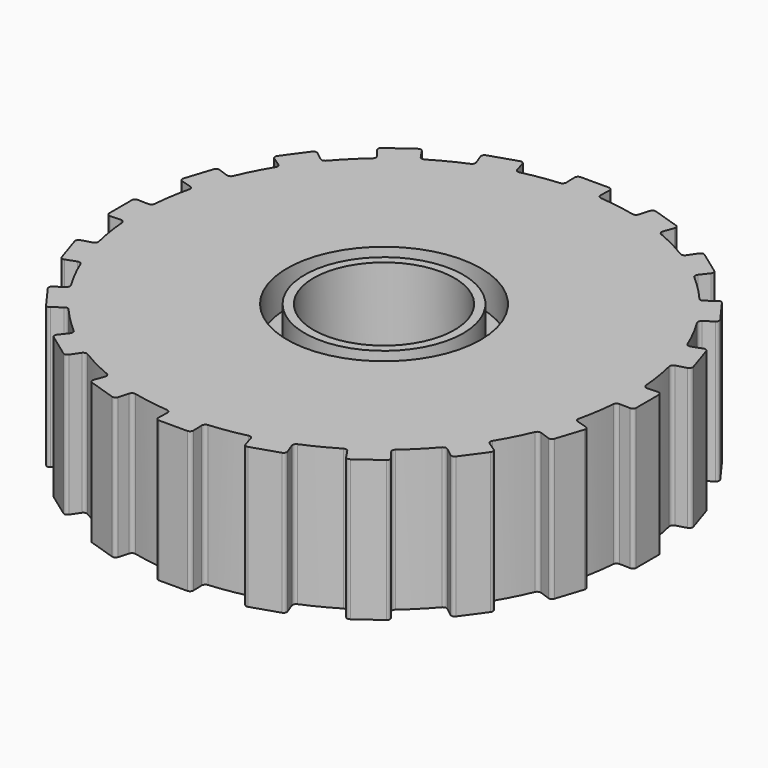
from build123d import *

# Parameters (mm, degrees)
F0_W     = 2.75
F0_H     = 2
F3_DEPTH = 25
F5_R     = 1.375
F5_R_2   = 1.125
F6_DEPTH = 0.5
F4_R     = 1.375
F4_R_2   = 1.125
F7_DEPTH = 0.5


with BuildPart() as f1:
    # F0 (on Front) → F1 (revolve)
    with BuildSketch(Plane.XZ):
        with Locations((-2.375, 1)):
            Rectangle(F0_W, F0_H)
    revolve(axis=Axis((0, 0, 1), (0, 0, 1)))

    # F2 (on face) → F3 (cut)
    with BuildSketch(Plane.XY.offset(2)):
        with BuildLine():
            ThreePointArc((-0.8032347269, 3.4065839155), (-0.5475206276, 3.4569091921), (-0.2887707016, 3.4880670122))
            Line((-0.2887707016, 3.4880670122), (-0.2983296172, 3.6916573868))
            Line((-0.2983296172, 3.6916573868), (-0.2483296172, 3.6916573868))
            Line((-0.2483296172, 3.6916573868), (-0.25, 3.7416573868))
            ThreePointArc((-0.25, 3.7416573868), (-0.5866292439, 3.7038312772), (-0.9184715906, 3.635781888))
            Line((-0.9184715906, 3.635781888), (-0.9046093693, 3.5877128856))
            Line((-0.9046093693, 3.5877128856), (-0.8630211073, 3.4435003366))
            ThreePointArc((-0.8630211073, 3.4435003366), (-0.8402539074, 3.4135015391), (-0.8032347269, 3.4065839155))
        make_face()
        with BuildLine():
            ThreePointArc((-0.2887707016, 3.4880670122), (-0.2557010319, 3.5060856191), (-0.2433182764, 3.5416516227))
            Line((-0.2433182764, 3.5416516227), (-0.2483296172, 3.6916573868))
            Line((-0.2483296172, 3.6916573868), (-0.2983296172, 3.6916573868))
            Line((-0.2983296172, 3.6916573868), (-0.2887707016, 3.4880670122))
        make_face()
        with BuildLine():
            ThreePointArc((-0.2483296172, 3.6916573868), (-0.2347697854, 3.7269080761), (-0.2, 3.7416573868))
            Line((-0.2, 3.7416573868), (-0.25, 3.7416573868))
            Line((-0.25, 3.7416573868), (-0.2483296172, 3.6916573868))
        make_face()
        with BuildLine():
            Line((-0.2, 3.7416573868), (0, 3.7416573868))
            Line((0, 3.7416573868), (0, 3.75))
            ThreePointArc((0, 3.75), (-0.1250695798, 3.7479137664), (-0.25, 3.7416573868))
            Line((-0.25, 3.7416573868), (-0.2, 3.7416573868))
        make_face()
        with BuildLine():
            Line((0, 3.75), (0, 3.7416573868))
            Line((0, 3.7416573868), (0.2, 3.7416573868))
            Line((0.2, 3.7416573868), (0.25, 3.7416573868))
            ThreePointArc((0.25, 3.7416573868), (0.1250695798, 3.7479137664), (0, 3.75))
        make_face()
        with BuildLine():
            Line((0.25, 3.7416573868), (0.2, 3.7416573868))
            ThreePointArc((0.2, 3.7416573868), (0.2347697854, 3.7269080761), (0.2483296172, 3.6916573868))
            Line((0.2483296172, 3.6916573868), (0.25, 3.7416573868))
        make_face()
        with BuildLine():
            Line((0.2983296172, 3.6916573868), (0.2887707016, 3.4880670122))
            ThreePointArc((0.2887707016, 3.4880670122), (0.5475206276, 3.4569091921), (0.8032347269, 3.4065839155))
            ThreePointArc((0.8032347269, 3.4065839155), (0.8402539074, 3.4135015391), (0.8630211073, 3.4435003366))
            Line((0.8630211073, 3.4435003366), (0.9046093693, 3.5877128856))
            Line((0.9046093693, 3.5877128856), (0.9184715906, 3.635781888))
            ThreePointArc((0.9184715906, 3.635781888), (0.5866292439, 3.7038312772), (0.25, 3.7416573868))
            Line((0.25, 3.7416573868), (0.2483296172, 3.6916573868))
            Line((0.2483296172, 3.6916573868), (0.2983296172, 3.6916573868))
        make_face()
        with BuildLine():
            Line((0.2483296172, 3.6916573868), (0.2433182764, 3.5416516227))
            ThreePointArc((0.2433182764, 3.5416516227), (0.2557010319, 3.5060856191), (0.2887707016, 3.4880670122))
            Line((0.2887707016, 3.4880670122), (0.2983296172, 3.6916573868))
            Line((0.2983296172, 3.6916573868), (0.2483296172, 3.6916573868))
        make_face()
        with BuildLine():
            Line((-2.8801181, -2.4015452797), (-2.8406490766, -2.370804649))
            ThreePointArc((-2.8406490766, -2.370804649), (-2.8771377525, -2.3805543499), (-2.9095073626, -2.36109443))
            Line((-2.9095073626, -2.36109443), (-2.8801181, -2.4015452797))
        make_face()
        with BuildLine():
            Line((-2.9095073626, -2.36109443), (-3.1446214635, -2.0374876322))
            Line((-3.1446214635, -2.0374876322), (-3.1740107261, -1.9970367825))
            ThreePointArc((-3.1740107261, -1.9970367825), (-3.0338137289, -2.2041946961), (-2.8801181, -2.4015452797))
            Line((-2.8801181, -2.4015452797), (-2.9095073626, -2.36109443))
        make_face()
        with BuildLine():
            ThreePointArc((-3.1446214635, -2.0374876322), (-3.1531261876, -2.0006888577), (-3.13257805, -1.9689988879))
            Line((-3.13257805, -1.9689988879), (-3.1740107261, -1.9970367825))
            Line((-3.1740107261, -1.9970367825), (-3.1446214635, -2.0374876322))
        make_face()
        with BuildLine():
            ThreePointArc((-2.9916406501, -1.8166139438), (-3.1185228347, -1.5889667491), (-3.228113807, -1.3525092417))
            ThreePointArc((-3.228113807, -1.3525092417), (-3.2554696104, -1.3266261727), (-3.2931213717, -1.3258399719))
            Line((-3.2931213717, -1.3258399719), (-3.4342367417, -1.3769603706))
            Line((-3.4342367417, -1.3769603706), (-3.4812733908, -1.3939998487))
            ThreePointArc((-3.4812733908, -1.3939998487), (-3.3412744657, -1.702464374), (-3.1740107261, -1.9970367825))
            Line((-3.1740107261, -1.9970367825), (-3.13257805, -1.9689988879))
            Line((-3.13257805, -1.9689988879), (-3.0082752454, -1.8848819719))
            ThreePointArc((-3.0082752454, -1.8848819719), (-2.9867801452, -1.8539589399), (-2.9916406501, -1.8166139438))
        make_face()
        with BuildLine():
            Line((-3.4812733908, -1.3939998487), (-3.4342367417, -1.3769603706))
            ThreePointArc((-3.4342367417, -1.3769603706), (-3.471952358, -1.3749572662), (-3.4967242406, -1.3464470229))
            Line((-3.4967242406, -1.3464470229), (-3.4812733908, -1.3939998487))
        make_face()
        with BuildLine():
            Line((-3.4967242406, -1.3464470229), (-3.6203310383, -0.9660244164))
            Line((-3.6203310383, -0.9660244164), (-3.635781888, -0.9184715906))
            ThreePointArc((-3.635781888, -0.9184715906), (-3.5664619361, -1.1588137289), (-3.4812733908, -1.3939998487))
            Line((-3.4812733908, -1.3939998487), (-3.4967242406, -1.3464470229))
        make_face()
        with BuildLine():
            ThreePointArc((-3.4065839155, -0.8032347269), (-3.4569091921, -0.5475206276), (-3.4880670122, -0.2887707016))
            ThreePointArc((-3.4880670122, -0.2887707016), (-3.5060856191, -0.2557010319), (-3.5416516227, -0.2433182764))
            Line((-3.5416516227, -0.2433182764), (-3.6916573868, -0.2483296172))
            Line((-3.6916573868, -0.2483296172), (-3.7416573868, -0.25))
            ThreePointArc((-3.7416573868, -0.25), (-3.7038312772, -0.5866292439), (-3.635781888, -0.9184715906))
            Line((-3.635781888, -0.9184715906), (-3.5877128856, -0.9046093693))
            Line((-3.5877128856, -0.9046093693), (-3.4435003366, -0.8630211073))
            ThreePointArc((-3.4435003366, -0.8630211073), (-3.4135015391, -0.8402539074), (-3.4065839155, -0.8032347269))
        make_face()
        with BuildLine():
            ThreePointArc((-3.6203310383, -0.9660244164), (-3.6170480649, -0.9283985978), (-3.5877128856, -0.9046093693))
            Line((-3.5877128856, -0.9046093693), (-3.635781888, -0.9184715906))
            Line((-3.635781888, -0.9184715906), (-3.6203310383, -0.9660244164))
        make_face()
        with BuildLine():
            Line((-3.7416573868, -0.2), (-3.7416573868, 0.2))
            Line((-3.7416573868, 0.2), (-3.7416573868, 0.25))
            ThreePointArc((-3.7416573868, 0.25), (-3.75, 0), (-3.7416573868, -0.25))
            Line((-3.7416573868, -0.25), (-3.7416573868, -0.2))
        make_face()
        with BuildLine():
            Line((-3.7416573868, -0.25), (-3.6916573868, -0.2483296172))
            ThreePointArc((-3.6916573868, -0.2483296172), (-3.7269080761, -0.2347697854), (-3.7416573868, -0.2))
            Line((-3.7416573868, -0.2), (-3.7416573868, -0.25))
        make_face()
        with BuildLine():
            ThreePointArc((-3.7416573868, 0.2), (-3.7269080761, 0.2347697854), (-3.6916573868, 0.2483296172))
            Line((-3.6916573868, 0.2483296172), (-3.7416573868, 0.25))
            Line((-3.7416573868, 0.25), (-3.7416573868, 0.2))
        make_face()
        with BuildLine():
            ThreePointArc((-3.4880670122, 0.2887707016), (-3.4569091921, 0.5475206276), (-3.4065839155, 0.8032347269))
            ThreePointArc((-3.4065839155, 0.8032347269), (-3.4135015391, 0.8402539074), (-3.4435003366, 0.8630211073))
            Line((-3.4435003366, 0.8630211073), (-3.5877128856, 0.9046093693))
            Line((-3.5877128856, 0.9046093693), (-3.635781888, 0.9184715906))
            ThreePointArc((-3.635781888, 0.9184715906), (-3.7038312772, 0.5866292439), (-3.7416573868, 0.25))
            Line((-3.7416573868, 0.25), (-3.6916573868, 0.2483296172))
            Line((-3.6916573868, 0.2483296172), (-3.5416516227, 0.2433182764))
            ThreePointArc((-3.5416516227, 0.2433182764), (-3.5060856191, 0.2557010319), (-3.4880670122, 0.2887707016))
        make_face()
        with BuildLine():
            Line((-3.635781888, 0.9184715906), (-3.5877128856, 0.9046093693))
            ThreePointArc((-3.5877128856, 0.9046093693), (-3.6170480649, 0.9283985978), (-3.6203310383, 0.9660244164))
            Line((-3.6203310383, 0.9660244164), (-3.635781888, 0.9184715906))
        make_face()
        with BuildLine():
            Line((-3.6203310383, 0.9660244164), (-3.4967242406, 1.3464470229))
            Line((-3.4967242406, 1.3464470229), (-3.4812733908, 1.3939998487))
            ThreePointArc((-3.4812733908, 1.3939998487), (-3.5664619361, 1.1588137289), (-3.635781888, 0.9184715906))
            Line((-3.635781888, 0.9184715906), (-3.6203310383, 0.9660244164))
        make_face()
        with BuildLine():
            ThreePointArc((-3.4967242406, 1.3464470229), (-3.471952358, 1.3749572662), (-3.4342367417, 1.3769603706))
            Line((-3.4342367417, 1.3769603706), (-3.4812733908, 1.3939998487))
            Line((-3.4812733908, 1.3939998487), (-3.4967242406, 1.3464470229))
        make_face()
        with BuildLine():
            ThreePointArc((-3.228113807, 1.3525092417), (-3.1185228347, 1.5889667491), (-2.9916406501, 1.8166139438))
            ThreePointArc((-2.9916406501, 1.8166139438), (-2.9867801452, 1.8539589399), (-3.0082752454, 1.8848819719))
            Line((-3.0082752454, 1.8848819719), (-3.13257805, 1.9689988879))
            Line((-3.13257805, 1.9689988879), (-3.1740107261, 1.9970367825))
            ThreePointArc((-3.1740107261, 1.9970367825), (-3.3412744657, 1.702464374), (-3.4812733908, 1.3939998487))
            Line((-3.4812733908, 1.3939998487), (-3.4342367417, 1.3769603706))
            Line((-3.4342367417, 1.3769603706), (-3.2931213717, 1.3258399719))
            ThreePointArc((-3.2931213717, 1.3258399719), (-3.2554696104, 1.3266261727), (-3.228113807, 1.3525092417))
        make_face()
        with BuildLine():
            Line((-3.1740107261, 1.9970367825), (-3.13257805, 1.9689988879))
            ThreePointArc((-3.13257805, 1.9689988879), (-3.1531261876, 2.0006888577), (-3.1446214635, 2.0374876322))
            Line((-3.1446214635, 2.0374876322), (-3.1740107261, 1.9970367825))
        make_face()
        with BuildLine():
            Line((-3.1446214635, 2.0374876322), (-2.9095073626, 2.36109443))
            Line((-2.9095073626, 2.36109443), (-2.8801181, 2.4015452797))
            ThreePointArc((-2.8801181, 2.4015452797), (-3.0338137289, 2.2041946961), (-3.1740107261, 1.9970367825))
            Line((-3.1740107261, 1.9970367825), (-3.1446214635, 2.0374876322))
        make_face()
        with BuildLine():
            ThreePointArc((-2.9095073626, 2.36109443), (-2.8771377525, 2.3805543499), (-2.8406490766, 2.370804649))
            Line((-2.8406490766, 2.370804649), (-2.8801181, 2.4015452797))
            Line((-2.8801181, 2.4015452797), (-2.9095073626, 2.36109443))
        make_face()
        with BuildLine():
            Line((-2.36109443, 2.9095073626), (-2.0374876322, 3.1446214635))
            Line((-2.0374876322, 3.1446214635), (-1.9970367825, 3.1740107261))
            ThreePointArc((-1.9970367825, 3.1740107261), (-2.2041946961, 3.0338137289), (-2.4015452797, 2.8801181))
            Line((-2.4015452797, 2.8801181), (-2.36109443, 2.9095073626))
        make_face()
        with BuildLine():
            Line((-2.4015452797, 2.8801181), (-2.370804649, 2.8406490766))
            ThreePointArc((-2.370804649, 2.8406490766), (-2.3805543499, 2.8771377525), (-2.36109443, 2.9095073626))
            Line((-2.36109443, 2.9095073626), (-2.4015452797, 2.8801181))
        make_face()
        with BuildLine():
            ThreePointArc((-2.6521703308, 2.2838547538), (-2.4748737342, 2.4748737342), (-2.2838547538, 2.6521703308))
            ThreePointArc((-2.2838547538, 2.6521703308), (-2.2676919005, 2.686185554), (-2.2785792132, 2.7222374564))
            Line((-2.2785792132, 2.7222374564), (-2.370804649, 2.8406490766))
            Line((-2.370804649, 2.8406490766), (-2.4015452797, 2.8801181))
            ThreePointArc((-2.4015452797, 2.8801181), (-2.6516504294, 2.6516504294), (-2.8801181, 2.4015452797))
            Line((-2.8801181, 2.4015452797), (-2.8406490766, 2.370804649))
            Line((-2.8406490766, 2.370804649), (-2.7222374564, 2.2785792132))
            ThreePointArc((-2.7222374564, 2.2785792132), (-2.686185554, 2.2676919005), (-2.6521703308, 2.2838547538))
        make_face()
        with BuildLine():
            ThreePointArc((-2.0374876322, 3.1446214635), (-2.0006888577, 3.1531261876), (-1.9689988879, 3.13257805))
            Line((-1.9689988879, 3.13257805), (-1.9970367825, 3.1740107261))
            Line((-1.9970367825, 3.1740107261), (-2.0374876322, 3.1446214635))
        make_face()
        with BuildLine():
            ThreePointArc((-1.8166139438, 2.9916406501), (-1.5889667491, 3.1185228347), (-1.3525092417, 3.228113807))
            ThreePointArc((-1.3525092417, 3.228113807), (-1.3266261727, 3.2554696104), (-1.3258399719, 3.2931213717))
            Line((-1.3258399719, 3.2931213717), (-1.3769603706, 3.4342367417))
            Line((-1.3769603706, 3.4342367417), (-1.3939998487, 3.4812733908))
            ThreePointArc((-1.3939998487, 3.4812733908), (-1.702464374, 3.3412744657), (-1.9970367825, 3.1740107261))
            Line((-1.9970367825, 3.1740107261), (-1.9689988879, 3.13257805))
            Line((-1.9689988879, 3.13257805), (-1.8848819719, 3.0082752454))
            ThreePointArc((-1.8848819719, 3.0082752454), (-1.8539589399, 2.9867801452), (-1.8166139438, 2.9916406501))
        make_face()
        with BuildLine():
            Line((-1.3939998487, 3.4812733908), (-1.3769603706, 3.4342367417))
            ThreePointArc((-1.3769603706, 3.4342367417), (-1.3749572662, 3.471952358), (-1.3464470229, 3.4967242406))
            Line((-1.3464470229, 3.4967242406), (-1.3939998487, 3.4812733908))
        make_face()
        with BuildLine():
            ThreePointArc((-0.9660244164, 3.6203310383), (-0.9283985978, 3.6170480649), (-0.9046093693, 3.5877128856))
            Line((-0.9046093693, 3.5877128856), (-0.9184715906, 3.635781888))
            Line((-0.9184715906, 3.635781888), (-0.9660244164, 3.6203310383))
        make_face()
        with BuildLine():
            Line((-0.9660244164, 3.6203310383), (-0.9184715906, 3.635781888))
            ThreePointArc((-0.9184715906, 3.635781888), (-1.1588137289, 3.5664619361), (-1.3939998487, 3.4812733908))
            Line((-1.3939998487, 3.4812733908), (-1.3464470229, 3.4967242406))
            Line((-1.3464470229, 3.4967242406), (-0.9660244164, 3.6203310383))
        make_face()
        with BuildLine():
            Line((3.1740107261, -1.9970367825), (3.13257805, -1.9689988879))
            ThreePointArc((3.13257805, -1.9689988879), (3.1531261876, -2.0006888577), (3.1446214635, -2.0374876322))
            Line((3.1446214635, -2.0374876322), (3.1740107261, -1.9970367825))
        make_face()
        with BuildLine():
            ThreePointArc((2.8801181, -2.4015452797), (3.0338137289, -2.2041946961), (3.1740107261, -1.9970367825))
            Line((3.1740107261, -1.9970367825), (3.1446214635, -2.0374876322))
            Line((3.1446214635, -2.0374876322), (2.9095073626, -2.36109443))
            Line((2.9095073626, -2.36109443), (2.8801181, -2.4015452797))
        make_face()
        with BuildLine():
            ThreePointArc((2.9095073626, -2.36109443), (2.8771377525, -2.3805543499), (2.8406490766, -2.370804649))
            Line((2.8406490766, -2.370804649), (2.8801181, -2.4015452797))
            Line((2.8801181, -2.4015452797), (2.9095073626, -2.36109443))
        make_face()
        with BuildLine():
            ThreePointArc((2.6521703308, -2.2838547538), (2.4748737342, -2.4748737342), (2.2838547538, -2.6521703308))
            ThreePointArc((2.2838547538, -2.6521703308), (2.2676919005, -2.686185554), (2.2785792132, -2.7222374564))
            Line((2.2785792132, -2.7222374564), (2.370804649, -2.8406490766))
            Line((2.370804649, -2.8406490766), (2.4015452797, -2.8801181))
            ThreePointArc((2.4015452797, -2.8801181), (2.6516504294, -2.6516504294), (2.8801181, -2.4015452797))
            Line((2.8801181, -2.4015452797), (2.8406490766, -2.370804649))
            Line((2.8406490766, -2.370804649), (2.7222374564, -2.2785792132))
            ThreePointArc((2.7222374564, -2.2785792132), (2.686185554, -2.2676919005), (2.6521703308, -2.2838547538))
        make_face()
        with BuildLine():
            Line((2.4015452797, -2.8801181), (2.370804649, -2.8406490766))
            ThreePointArc((2.370804649, -2.8406490766), (2.3805543499, -2.8771377525), (2.36109443, -2.9095073626))
            Line((2.36109443, -2.9095073626), (2.4015452797, -2.8801181))
        make_face()
        with BuildLine():
            ThreePointArc((1.9970367825, -3.1740107261), (2.2041946961, -3.0338137289), (2.4015452797, -2.8801181))
            Line((2.4015452797, -2.8801181), (2.36109443, -2.9095073626))
            Line((2.36109443, -2.9095073626), (2.0374876322, -3.1446214635))
            Line((2.0374876322, -3.1446214635), (1.9970367825, -3.1740107261))
        make_face()
        with BuildLine():
            ThreePointArc((2.0374876322, -3.1446214635), (2.0006888577, -3.1531261876), (1.9689988879, -3.13257805))
            Line((1.9689988879, -3.13257805), (1.9970367825, -3.1740107261))
            Line((1.9970367825, -3.1740107261), (2.0374876322, -3.1446214635))
        make_face()
        with BuildLine():
            ThreePointArc((1.8166139438, -2.9916406501), (1.5889667491, -3.1185228347), (1.3525092417, -3.228113807))
            ThreePointArc((1.3525092417, -3.228113807), (1.3266261727, -3.2554696104), (1.3258399719, -3.2931213717))
            Line((1.3258399719, -3.2931213717), (1.3769603706, -3.4342367417))
            Line((1.3769603706, -3.4342367417), (1.3939998487, -3.4812733908))
            ThreePointArc((1.3939998487, -3.4812733908), (1.702464374, -3.3412744657), (1.9970367825, -3.1740107261))
            Line((1.9970367825, -3.1740107261), (1.9689988879, -3.13257805))
            Line((1.9689988879, -3.13257805), (1.8848819719, -3.0082752454))
            ThreePointArc((1.8848819719, -3.0082752454), (1.8539589399, -2.9867801452), (1.8166139438, -2.9916406501))
        make_face()
        with BuildLine():
            Line((1.3939998487, -3.4812733908), (1.3769603706, -3.4342367417))
            ThreePointArc((1.3769603706, -3.4342367417), (1.3749572662, -3.471952358), (1.3464470229, -3.4967242406))
            Line((1.3464470229, -3.4967242406), (1.3939998487, -3.4812733908))
        make_face()
        with BuildLine():
            ThreePointArc((0.9184715906, -3.635781888), (1.1588137289, -3.5664619361), (1.3939998487, -3.4812733908))
            Line((1.3939998487, -3.4812733908), (1.3464470229, -3.4967242406))
            Line((1.3464470229, -3.4967242406), (0.9660244164, -3.6203310383))
            Line((0.9660244164, -3.6203310383), (0.9184715906, -3.635781888))
        make_face()
        with BuildLine():
            Line((0.25, -3.7416573868), (0.2483296172, -3.6916573868))
            ThreePointArc((0.2483296172, -3.6916573868), (0.2347697854, -3.7269080761), (0.2, -3.7416573868))
            Line((0.2, -3.7416573868), (0.25, -3.7416573868))
        make_face()
        with BuildLine():
            ThreePointArc((-0.25, -3.7416573868), (0, -3.75), (0.25, -3.7416573868))
            Line((0.25, -3.7416573868), (0.2, -3.7416573868))
            Line((0.2, -3.7416573868), (-0.2, -3.7416573868))
            Line((-0.2, -3.7416573868), (-0.25, -3.7416573868))
        make_face()
        with BuildLine():
            Line((-0.9184715906, -3.635781888), (-0.9046093693, -3.5877128856))
            ThreePointArc((-0.9046093693, -3.5877128856), (-0.9283985978, -3.6170480649), (-0.9660244164, -3.6203310383))
            Line((-0.9660244164, -3.6203310383), (-0.9184715906, -3.635781888))
        make_face()
        with BuildLine():
            Line((-0.9660244164, -3.6203310383), (-1.3464470229, -3.4967242406))
            Line((-1.3464470229, -3.4967242406), (-1.3939998487, -3.4812733908))
            ThreePointArc((-1.3939998487, -3.4812733908), (-1.1588137289, -3.5664619361), (-0.9184715906, -3.635781888))
            Line((-0.9184715906, -3.635781888), (-0.9660244164, -3.6203310383))
        make_face()
        with BuildLine():
            ThreePointArc((-1.3464470229, -3.4967242406), (-1.3749572662, -3.471952358), (-1.3769603706, -3.4342367417))
            Line((-1.3769603706, -3.4342367417), (-1.3939998487, -3.4812733908))
            Line((-1.3939998487, -3.4812733908), (-1.3464470229, -3.4967242406))
        make_face()
        with BuildLine():
            ThreePointArc((-1.3525092417, -3.228113807), (-1.5889667491, -3.1185228347), (-1.8166139438, -2.9916406501))
            ThreePointArc((-1.8166139438, -2.9916406501), (-1.8539589399, -2.9867801452), (-1.8848819719, -3.0082752454))
            Line((-1.8848819719, -3.0082752454), (-1.9689988879, -3.13257805))
            Line((-1.9689988879, -3.13257805), (-1.9970367825, -3.1740107261))
            ThreePointArc((-1.9970367825, -3.1740107261), (-1.702464374, -3.3412744657), (-1.3939998487, -3.4812733908))
            Line((-1.3939998487, -3.4812733908), (-1.3769603706, -3.4342367417))
            Line((-1.3769603706, -3.4342367417), (-1.3258399719, -3.2931213717))
            ThreePointArc((-1.3258399719, -3.2931213717), (-1.3266261727, -3.2554696104), (-1.3525092417, -3.228113807))
        make_face()
        with BuildLine():
            ThreePointArc((-0.2887707016, -3.4880670122), (-0.5475206276, -3.4569091921), (-0.8032347269, -3.4065839155))
            ThreePointArc((-0.8032347269, -3.4065839155), (-0.8402539074, -3.4135015391), (-0.8630211073, -3.4435003366))
            Line((-0.8630211073, -3.4435003366), (-0.9046093693, -3.5877128856))
            Line((-0.9046093693, -3.5877128856), (-0.9184715906, -3.635781888))
            ThreePointArc((-0.9184715906, -3.635781888), (-0.5866292439, -3.7038312772), (-0.25, -3.7416573868))
            Line((-0.25, -3.7416573868), (-0.2483296172, -3.6916573868))
            Line((-0.2483296172, -3.6916573868), (-0.2433182764, -3.5416516227))
            ThreePointArc((-0.2433182764, -3.5416516227), (-0.2557010319, -3.5060856191), (-0.2887707016, -3.4880670122))
        make_face()
        with BuildLine():
            ThreePointArc((0.8032347269, -3.4065839155), (0.5475206276, -3.4569091921), (0.2887707016, -3.4880670122))
            ThreePointArc((0.2887707016, -3.4880670122), (0.2557010319, -3.5060856191), (0.2433182764, -3.5416516227))
            Line((0.2433182764, -3.5416516227), (0.2483296172, -3.6916573868))
            Line((0.2483296172, -3.6916573868), (0.25, -3.7416573868))
            ThreePointArc((0.25, -3.7416573868), (0.5866292439, -3.7038312772), (0.9184715906, -3.635781888))
            Line((0.9184715906, -3.635781888), (0.9046093693, -3.5877128856))
            Line((0.9046093693, -3.5877128856), (0.8630211073, -3.4435003366))
            ThreePointArc((0.8630211073, -3.4435003366), (0.8402539074, -3.4135015391), (0.8032347269, -3.4065839155))
        make_face()
        with BuildLine():
            ThreePointArc((-0.2, -3.7416573868), (-0.2347697854, -3.7269080761), (-0.2483296172, -3.6916573868))
            Line((-0.2483296172, -3.6916573868), (-0.25, -3.7416573868))
            Line((-0.25, -3.7416573868), (-0.2, -3.7416573868))
        make_face()
        with BuildLine():
            ThreePointArc((0.9660244164, -3.6203310383), (0.9283985978, -3.6170480649), (0.9046093693, -3.5877128856))
            Line((0.9046093693, -3.5877128856), (0.9184715906, -3.635781888))
            Line((0.9184715906, -3.635781888), (0.9660244164, -3.6203310383))
        make_face()
        with BuildLine():
            Line((-1.9970367825, -3.1740107261), (-1.9689988879, -3.13257805))
            ThreePointArc((-1.9689988879, -3.13257805), (-2.0006888577, -3.1531261876), (-2.0374876322, -3.1446214635))
            Line((-2.0374876322, -3.1446214635), (-1.9970367825, -3.1740107261))
        make_face()
        with BuildLine():
            Line((-2.0374876322, -3.1446214635), (-2.36109443, -2.9095073626))
            Line((-2.36109443, -2.9095073626), (-2.4015452797, -2.8801181))
            ThreePointArc((-2.4015452797, -2.8801181), (-2.2041946961, -3.0338137289), (-1.9970367825, -3.1740107261))
            Line((-1.9970367825, -3.1740107261), (-2.0374876322, -3.1446214635))
        make_face()
        with BuildLine():
            ThreePointArc((-2.36109443, -2.9095073626), (-2.3805543499, -2.8771377525), (-2.370804649, -2.8406490766))
            Line((-2.370804649, -2.8406490766), (-2.4015452797, -2.8801181))
            Line((-2.4015452797, -2.8801181), (-2.36109443, -2.9095073626))
        make_face()
        with BuildLine():
            ThreePointArc((-2.2838547538, -2.6521703308), (-2.4748737342, -2.4748737342), (-2.6521703308, -2.2838547538))
            ThreePointArc((-2.6521703308, -2.2838547538), (-2.686185554, -2.2676919005), (-2.7222374564, -2.2785792132))
            Line((-2.7222374564, -2.2785792132), (-2.8406490766, -2.370804649))
            Line((-2.8406490766, -2.370804649), (-2.8801181, -2.4015452797))
            ThreePointArc((-2.8801181, -2.4015452797), (-2.6516504294, -2.6516504294), (-2.4015452797, -2.8801181))
            Line((-2.4015452797, -2.8801181), (-2.370804649, -2.8406490766))
            Line((-2.370804649, -2.8406490766), (-2.2785792132, -2.7222374564))
            ThreePointArc((-2.2785792132, -2.7222374564), (-2.2676919005, -2.686185554), (-2.2838547538, -2.6521703308))
        make_face()
        with BuildLine():
            ThreePointArc((3.228113807, -1.3525092417), (3.1185228347, -1.5889667491), (2.9916406501, -1.8166139438))
            ThreePointArc((2.9916406501, -1.8166139438), (2.9867801452, -1.8539589399), (3.0082752454, -1.8848819719))
            Line((3.0082752454, -1.8848819719), (3.13257805, -1.9689988879))
            Line((3.13257805, -1.9689988879), (3.1740107261, -1.9970367825))
            ThreePointArc((3.1740107261, -1.9970367825), (3.3412744657, -1.702464374), (3.4812733908, -1.3939998487))
            Line((3.4812733908, -1.3939998487), (3.4342367417, -1.3769603706))
            Line((3.4342367417, -1.3769603706), (3.2931213717, -1.3258399719))
            ThreePointArc((3.2931213717, -1.3258399719), (3.2554696104, -1.3266261727), (3.228113807, -1.3525092417))
        make_face()
        with BuildLine():
            ThreePointArc((3.4967242406, -1.3464470229), (3.471952358, -1.3749572662), (3.4342367417, -1.3769603706))
            Line((3.4342367417, -1.3769603706), (3.4812733908, -1.3939998487))
            Line((3.4812733908, -1.3939998487), (3.4967242406, -1.3464470229))
        make_face()
        with BuildLine():
            ThreePointArc((3.4812733908, -1.3939998487), (3.5664619361, -1.1588137289), (3.635781888, -0.9184715906))
            Line((3.635781888, -0.9184715906), (3.6203310383, -0.9660244164))
            Line((3.6203310383, -0.9660244164), (3.4967242406, -1.3464470229))
            Line((3.4967242406, -1.3464470229), (3.4812733908, -1.3939998487))
        make_face()
        with BuildLine():
            Line((3.635781888, -0.9184715906), (3.5877128856, -0.9046093693))
            ThreePointArc((3.5877128856, -0.9046093693), (3.6170480649, -0.9283985978), (3.6203310383, -0.9660244164))
            Line((3.6203310383, -0.9660244164), (3.635781888, -0.9184715906))
        make_face()
        with BuildLine():
            ThreePointArc((3.4880670122, -0.2887707016), (3.4569091921, -0.5475206276), (3.4065839155, -0.8032347269))
            ThreePointArc((3.4065839155, -0.8032347269), (3.4135015391, -0.8402539074), (3.4435003366, -0.8630211073))
            Line((3.4435003366, -0.8630211073), (3.5877128856, -0.9046093693))
            Line((3.5877128856, -0.9046093693), (3.635781888, -0.9184715906))
            ThreePointArc((3.635781888, -0.9184715906), (3.7038312772, -0.5866292439), (3.7416573868, -0.25))
            Line((3.7416573868, -0.25), (3.6916573868, -0.2483296172))
            Line((3.6916573868, -0.2483296172), (3.5416516227, -0.2433182764))
            ThreePointArc((3.5416516227, -0.2433182764), (3.5060856191, -0.2557010319), (3.4880670122, -0.2887707016))
        make_face()
        with BuildLine():
            ThreePointArc((3.75, 0), (3.7479137664, 0.1250695798), (3.7416573868, 0.25))
            Line((3.7416573868, 0.25), (3.7416573868, 0.2))
            Line((3.7416573868, 0.2), (3.7416573868, -0.2))
            Line((3.7416573868, -0.2), (3.7416573868, -0.25))
            ThreePointArc((3.7416573868, -0.25), (3.7479137664, -0.1250695798), (3.75, 0))
        make_face()
        with BuildLine():
            Line((3.7416573868, 0.25), (3.6916573868, 0.2483296172))
            ThreePointArc((3.6916573868, 0.2483296172), (3.7269080761, 0.2347697854), (3.7416573868, 0.2))
            Line((3.7416573868, 0.2), (3.7416573868, 0.25))
        make_face()
        with BuildLine():
            ThreePointArc((3.7416573868, -0.2), (3.7269080761, -0.2347697854), (3.6916573868, -0.2483296172))
            Line((3.6916573868, -0.2483296172), (3.7416573868, -0.25))
            Line((3.7416573868, -0.25), (3.7416573868, -0.2))
        make_face()
        with BuildLine():
            ThreePointArc((3.4065839155, 0.8032347269), (3.4569091921, 0.5475206276), (3.4880670122, 0.2887707016))
            ThreePointArc((3.4880670122, 0.2887707016), (3.5060856191, 0.2557010319), (3.5416516227, 0.2433182764))
            Line((3.5416516227, 0.2433182764), (3.6916573868, 0.2483296172))
            Line((3.6916573868, 0.2483296172), (3.7416573868, 0.25))
            ThreePointArc((3.7416573868, 0.25), (3.7038312772, 0.5866292439), (3.635781888, 0.9184715906))
            Line((3.635781888, 0.9184715906), (3.5877128856, 0.9046093693))
            Line((3.5877128856, 0.9046093693), (3.4435003366, 0.8630211073))
            ThreePointArc((3.4435003366, 0.8630211073), (3.4135015391, 0.8402539074), (3.4065839155, 0.8032347269))
        make_face()
        with BuildLine():
            ThreePointArc((3.6203310383, 0.9660244164), (3.6170480649, 0.9283985978), (3.5877128856, 0.9046093693))
            Line((3.5877128856, 0.9046093693), (3.635781888, 0.9184715906))
            Line((3.635781888, 0.9184715906), (3.6203310383, 0.9660244164))
        make_face()
        with BuildLine():
            ThreePointArc((3.635781888, 0.9184715906), (3.5664619361, 1.1588137289), (3.4812733908, 1.3939998487))
            Line((3.4812733908, 1.3939998487), (3.4967242406, 1.3464470229))
            Line((3.4967242406, 1.3464470229), (3.6203310383, 0.9660244164))
            Line((3.6203310383, 0.9660244164), (3.635781888, 0.9184715906))
        make_face()
        with BuildLine():
            Line((3.4812733908, 1.3939998487), (3.4342367417, 1.3769603706))
            ThreePointArc((3.4342367417, 1.3769603706), (3.471952358, 1.3749572662), (3.4967242406, 1.3464470229))
            Line((3.4967242406, 1.3464470229), (3.4812733908, 1.3939998487))
        make_face()
        with BuildLine():
            ThreePointArc((2.9916406501, 1.8166139438), (3.1185228347, 1.5889667491), (3.228113807, 1.3525092417))
            ThreePointArc((3.228113807, 1.3525092417), (3.2554696104, 1.3266261727), (3.2931213717, 1.3258399719))
            Line((3.2931213717, 1.3258399719), (3.4342367417, 1.3769603706))
            Line((3.4342367417, 1.3769603706), (3.4812733908, 1.3939998487))
            ThreePointArc((3.4812733908, 1.3939998487), (3.3412744657, 1.702464374), (3.1740107261, 1.9970367825))
            Line((3.1740107261, 1.9970367825), (3.13257805, 1.9689988879))
            Line((3.13257805, 1.9689988879), (3.0082752454, 1.8848819719))
            ThreePointArc((3.0082752454, 1.8848819719), (2.9867801452, 1.8539589399), (2.9916406501, 1.8166139438))
        make_face()
        with BuildLine():
            ThreePointArc((3.1740107261, 1.9970367825), (3.0338137289, 2.2041946961), (2.8801181, 2.4015452797))
            Line((2.8801181, 2.4015452797), (2.9095073626, 2.36109443))
            Line((2.9095073626, 2.36109443), (3.1446214635, 2.0374876322))
            Line((3.1446214635, 2.0374876322), (3.1740107261, 1.9970367825))
        make_face()
        with BuildLine():
            ThreePointArc((3.1446214635, 2.0374876322), (3.1531261876, 2.0006888577), (3.13257805, 1.9689988879))
            Line((3.13257805, 1.9689988879), (3.1740107261, 1.9970367825))
            Line((3.1740107261, 1.9970367825), (3.1446214635, 2.0374876322))
        make_face()
        with BuildLine():
            Line((2.8801181, 2.4015452797), (2.8406490766, 2.370804649))
            ThreePointArc((2.8406490766, 2.370804649), (2.8771377525, 2.3805543499), (2.9095073626, 2.36109443))
            Line((2.9095073626, 2.36109443), (2.8801181, 2.4015452797))
        make_face()
        with BuildLine():
            ThreePointArc((2.2785792132, 2.7222374564), (2.2676919005, 2.686185554), (2.2838547538, 2.6521703308))
            ThreePointArc((2.2838547538, 2.6521703308), (2.4748737342, 2.4748737342), (2.6521703308, 2.2838547538))
            ThreePointArc((2.6521703308, 2.2838547538), (2.686185554, 2.2676919005), (2.7222374564, 2.2785792132))
            Line((2.7222374564, 2.2785792132), (2.8406490766, 2.370804649))
            Line((2.8406490766, 2.370804649), (2.8801181, 2.4015452797))
            ThreePointArc((2.8801181, 2.4015452797), (2.6516504294, 2.6516504294), (2.4015452797, 2.8801181))
            Line((2.4015452797, 2.8801181), (2.370804649, 2.8406490766))
            Line((2.370804649, 2.8406490766), (2.2785792132, 2.7222374564))
        make_face()
        with BuildLine():
            ThreePointArc((2.4015452797, 2.8801181), (2.2041946961, 3.0338137289), (1.9970367825, 3.1740107261))
            Line((1.9970367825, 3.1740107261), (2.0374876322, 3.1446214635))
            Line((2.0374876322, 3.1446214635), (2.36109443, 2.9095073626))
            Line((2.36109443, 2.9095073626), (2.4015452797, 2.8801181))
        make_face()
        with BuildLine():
            ThreePointArc((2.36109443, 2.9095073626), (2.3805543499, 2.8771377525), (2.370804649, 2.8406490766))
            Line((2.370804649, 2.8406490766), (2.4015452797, 2.8801181))
            Line((2.4015452797, 2.8801181), (2.36109443, 2.9095073626))
        make_face()
        with BuildLine():
            ThreePointArc((1.3939998487, 3.4812733908), (1.1588137289, 3.5664619361), (0.9184715906, 3.635781888))
            Line((0.9184715906, 3.635781888), (0.9660244164, 3.6203310383))
            Line((0.9660244164, 3.6203310383), (1.3464470229, 3.4967242406))
            Line((1.3464470229, 3.4967242406), (1.3939998487, 3.4812733908))
        make_face()
        with BuildLine():
            ThreePointArc((1.3464470229, 3.4967242406), (1.3749572662, 3.471952358), (1.3769603706, 3.4342367417))
            Line((1.3769603706, 3.4342367417), (1.3939998487, 3.4812733908))
            Line((1.3939998487, 3.4812733908), (1.3464470229, 3.4967242406))
        make_face()
        with BuildLine():
            Line((0.9184715906, 3.635781888), (0.9046093693, 3.5877128856))
            ThreePointArc((0.9046093693, 3.5877128856), (0.9283985978, 3.6170480649), (0.9660244164, 3.6203310383))
            Line((0.9660244164, 3.6203310383), (0.9184715906, 3.635781888))
        make_face()
        with BuildLine():
            ThreePointArc((1.3258399719, 3.2931213717), (1.3266261727, 3.2554696104), (1.3525092417, 3.228113807))
            ThreePointArc((1.3525092417, 3.228113807), (1.5889667491, 3.1185228347), (1.8166139438, 2.9916406501))
            ThreePointArc((1.8166139438, 2.9916406501), (1.8539589399, 2.9867801452), (1.8848819719, 3.0082752454))
            Line((1.8848819719, 3.0082752454), (1.9689988879, 3.13257805))
            Line((1.9689988879, 3.13257805), (1.9970367825, 3.1740107261))
            ThreePointArc((1.9970367825, 3.1740107261), (1.702464374, 3.3412744657), (1.3939998487, 3.4812733908))
            Line((1.3939998487, 3.4812733908), (1.3769603706, 3.4342367417))
            Line((1.3769603706, 3.4342367417), (1.3258399719, 3.2931213717))
        make_face()
        with BuildLine():
            Line((1.9970367825, 3.1740107261), (1.9689988879, 3.13257805))
            ThreePointArc((1.9689988879, 3.13257805), (2.0006888577, 3.1531261876), (2.0374876322, 3.1446214635))
            Line((2.0374876322, 3.1446214635), (1.9970367825, 3.1740107261))
        make_face()
    extrude(amount=-F3_DEPTH, mode=Mode.SUBTRACT)

    # F5 (on face) → F6 (cut)
    with BuildSketch(Plane(origin=(0, 0, 0), x_dir=(1, 0, 0), z_dir=(0, 0, -1))):
        Circle(F5_R)
        Circle(F5_R_2, mode=Mode.SUBTRACT)
    extrude(amount=-F6_DEPTH, mode=Mode.SUBTRACT)

    # F4 (on face) → F7 (cut)
    with BuildSketch(Plane.XY.offset(2)):
        Circle(F4_R)
        Circle(F4_R_2, mode=Mode.SUBTRACT)
    extrude(amount=-F7_DEPTH, mode=Mode.SUBTRACT)


solid = f1.part
